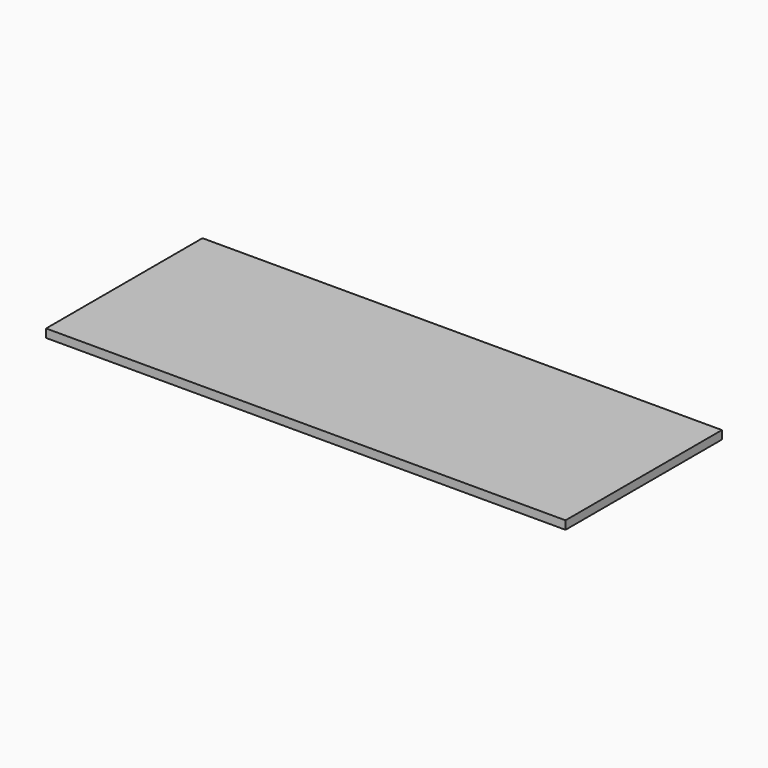
from build123d import *

# Parameters (mm, degrees)
F0_W     = 1181.1
F0_H     = 444.5
F1_DEPTH = 19.05


# Not quite as in the source:
# - a length typed as a fraction of an inch, garbled in the dataset ("3 / 203.2 mm" for 3/8 in), is restored


with BuildPart() as f1:
    # F0 (on Top) → F1 (new body)
    with BuildSketch(Plane.XY):
        with Locations((0, 222.25)):
            Rectangle(F0_W, F0_H)
    extrude(amount=F1_DEPTH)


solid = f1.part
